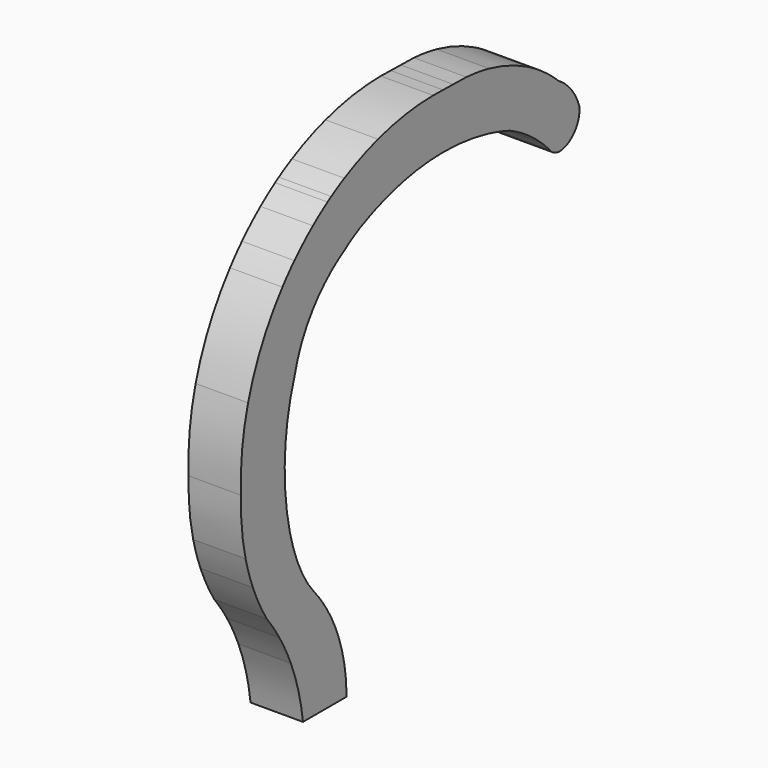
from build123d import *

# Parameters (mm, degrees)
F0_W     = 7.3179761397
F0_H     = 0.852221109
F2_DEPTH = 8


with BuildPart() as f2:
    # F0 (on Right) → F2 (new body)
    with BuildSketch(Plane.YZ):
        with BuildLine():
            Line((-10.1888944263, 53.9168607201), (-5.7503742038, 53.9168607201))
            ThreePointArc((-5.7503742038, 53.9168607201), (-4.3894384073, 57.8607093725), (-2.2639043723, 61.4507223949))
            Line((-2.2639043723, 61.4507223949), (-2.2639043723, 66.7907201963))
            add(Edge.make_bspline(
                [(-10.1888944263, 53.9168607201), (-8.3345715025, 58.6916164824), (-4.5405432149, 63.9948893867), (-2.2639043723, 66.7907201963)],
                knots=[0.4485191098, 0.4485191098, 0.4485191098, 0.4485191098, 0.5436368318, 0.5436368318, 0.5436368318, 0.5436368318], degree=3))
        make_face()
        with BuildLine():
            add(Edge.make_bspline(
                [(-5.7503742038, 53.9168607201), (-7.6414888716, 48.4947767316), (-7.6414888716, 42.0372994525)],
                knots=[4.1382491567, 4.1382491567, 4.1382491567, 4.7123889804, 4.7123889804, 4.7123889804], degree=2, weights=[1, 0.9590776261, 1]))
            Line((-5.7503742038, 53.9168607201), (-10.1888944263, 53.9168607201))
            add(Edge.make_bspline(
                [(-11.7964888716, 42.0372994525), (-11.953273607, 45.832214532), (-11.8401507048, 49.6649877966), (-10.1888944263, 53.9168607201)],
                knots=[0.3638177163, 0.3638177163, 0.3638177163, 0.3638177163, 0.4485191098, 0.4485191098, 0.4485191098, 0.4485191098], degree=3))
            Line((-11.7964888716, 42.0372994525), (-7.6414888716, 42.0372994525))
        make_face()
        with BuildLine():
            add(Edge.make_bspline(
                [(-7.6414888716, 42.0372994525), (-7.6414888716, 37.3930199427), (-6.6239046752, 33.1494348573)],
                knots=[4.7123889804, 4.7123889804, 4.7123889804, 5.1308312404, 5.1308312404, 5.1308312404], degree=2, weights=[1, 0.9781929812, 1]))
            Line((-7.6414888716, 42.0372994525), (-11.7964888716, 42.0372994525))
            add(Edge.make_bspline(
                [(-10.8578113303, 33.1494348573), (-11.3245159446, 35.5121547718), (-11.6611145328, 38.7606149052), (-11.7964888716, 42.0372994525)],
                knots=[0.2906830765, 0.2906830765, 0.2906830765, 0.2906830765, 0.3638177163, 0.3638177163, 0.3638177163, 0.3638177163], degree=3))
            Line((-10.8578113303, 33.1494348573), (-6.6239046752, 33.1494348573))
        make_face()
        with BuildLine():
            Line((-2.2639043723, 66.7907201963), (-2.2639043723, 61.4507223949))
            ThreePointArc((-2.2639043723, 61.4507223949), (-0.6270073096, 63.4042822038), (1.237973472, 65.1414277376))
            Line((1.237973472, 65.1414277376), (1.237973472, 66.7907201963))
            Line((1.237973472, 66.7907201963), (-2.2639043723, 66.7907201963))
        make_face()
        with BuildLine():
            add(Edge.make_bspline(
                [(-11.7964888716, 42.0372994525), (-11.953273607, 45.832214532), (-11.8401507048, 49.6649877966), (-10.1888944263, 53.9168607201)],
                knots=[0.3638177163, 0.3638177163, 0.3638177163, 0.3638177163, 0.4485191098, 0.4485191098, 0.4485191098, 0.4485191098], degree=3))
            Line((-10.1888944263, 53.9168607201), (-14.6274146488, 53.9168607201))
            ThreePointArc((-14.6274146488, 53.9168607201), (-15.7735164452, 48.0310330528), (-15.9514888716, 42.0372994525))
            Line((-15.9514888716, 42.0372994525), (-11.7964888716, 42.0372994525))
        make_face()
        with BuildLine():
            Line((-14.6274146488, 53.9168607201), (-10.1888944263, 53.9168607201))
            add(Edge.make_bspline(
                [(-10.1888944263, 53.9168607201), (-8.3345715025, 58.6916164824), (-4.5405432149, 63.9948893867), (-2.2639043723, 66.7907201963)],
                knots=[0.4485191098, 0.4485191098, 0.4485191098, 0.4485191098, 0.5436368318, 0.5436368318, 0.5436368318, 0.5436368318], degree=3))
            Line((-2.2639043723, 66.7907201963), (-8.0789732143, 66.7907201963))
            ThreePointArc((-8.0789732143, 66.7907201963), (-11.9890354693, 60.6772188038), (-14.6274146488, 53.9168607201))
        make_face()
        with BuildLine():
            add(Edge.make_bspline(
                [(-6.6239046752, 33.1494348573), (-6.0548250045, 30.7762277933), (-5.2018884672, 28.7161691389)],
                knots=[5.1308312404, 5.1308312404, 5.1308312404, 5.3672118342, 5.3672118342, 5.3672118342], degree=2, weights=[1, 0.9930236536, 1]))
            Line((-6.6239046752, 33.1494348573), (-10.8578113303, 33.1494348573))
            add(Edge.make_bspline(
                [(-9.4522823352, 28.7161691389), (-10.1167744763, 30.2015624686), (-10.5211448069, 31.4450405251), (-10.8578113303, 33.1494348573)],
                knots=[0.2379259703, 0.2379259703, 0.2379259703, 0.2379259703, 0.2906830765, 0.2906830765, 0.2906830765, 0.2906830765], degree=3))
            Line((-9.4522823352, 28.7161691389), (-5.2018884672, 28.7161691389))
        make_face()
        with BuildLine():
            add(Edge.make_bspline(
                [(-10.8578113303, 33.1494348573), (-11.3245159446, 35.5121547718), (-11.6611145328, 38.7606149052), (-11.7964888716, 42.0372994525)],
                knots=[0.2906830765, 0.2906830765, 0.2906830765, 0.2906830765, 0.3638177163, 0.3638177163, 0.3638177163, 0.3638177163], degree=3))
            Line((-11.7964888716, 42.0372994525), (-15.9514888716, 42.0372994525))
            ThreePointArc((-15.9514888716, 42.0372994525), (-15.825139965, 37.5640044352), (-15.0917179854, 33.1494348573))
            Line((-15.0917179854, 33.1494348573), (-10.8578113303, 33.1494348573))
        make_face()
        with BuildLine():
            Line((1.237973472, 66.7907201963), (1.237973472, 65.1414277376))
            ThreePointArc((1.237973472, 65.1414277376), (2.366186126, 66.0058819106), (3.5511644697, 66.7907201963))
            Line((3.5511644697, 66.7907201963), (1.237973472, 66.7907201963))
        make_face()
        with BuildLine():
            add(Edge.make_bspline(
                [(-2.2639043723, 66.7907201963), (-1.2992613055, 67.9753520122), (-0.6070401721, 68.7098144761), (0.2691752969, 69.4241264728)],
                knots=[0.5436368318, 0.5436368318, 0.5436368318, 0.5436368318, 0.5839395136, 0.5839395136, 0.5839395136, 0.5839395136], degree=3))
            Line((-2.2639043723, 66.7907201963), (1.237973472, 66.7907201963))
            Line((1.237973472, 66.7907201963), (1.237973472, 69.4241264728))
            Line((1.237973472, 69.4241264728), (0.2691752969, 69.4241264728))
        make_face()
        with BuildLine():
            Line((-8.0789732143, 66.7907201963), (-2.2639043723, 66.7907201963))
            Line((-2.2639043723, 66.7907201963), (-2.2639043723, 69.4241264728))
            Line((-2.2639043723, 69.4241264728), (-5.7937727942, 69.4241264728))
            ThreePointArc((-5.7937727942, 69.4241264728), (-6.9674844154, 68.1344209955), (-8.0789732143, 66.7907201963))
        make_face()
        with BuildLine():
            Line((-2.2639043723, 69.4241264728), (-2.2639043723, 66.7907201963))
            add(Edge.make_bspline(
                [(-2.2639043723, 66.7907201963), (-1.2992613055, 67.9753520122), (-0.6070401721, 68.7098144761), (0.2691752969, 69.4241264728)],
                knots=[0.5436368318, 0.5436368318, 0.5436368318, 0.5436368318, 0.5839395136, 0.5839395136, 0.5839395136, 0.5839395136], degree=3))
            Line((0.2691752969, 69.4241264728), (-2.2639043723, 69.4241264728))
        make_face()
        with BuildLine():
            add(Edge.make_bspline(
                [(-5.2018884672, 28.7161691389), (-3.8937096158, 25.55658452), (-2.0688837208, 23.4551739871)],
                knots=[5.3672118342, 5.3672118342, 5.3672118342, 5.727505896, 5.727505896, 5.727505896], degree=2, weights=[1, 0.9838173593, 1]))
            Line((-5.2018884672, 28.7161691389), (-9.4522823352, 28.7161691389))
            add(Edge.make_bspline(
                [(-6.5688837208, 23.4551739871), (-7.6073097342, 25.0299710332), (-8.6975714446, 27.0291025005), (-9.4522823352, 28.7161691389)],
                knots=[0.1780059801, 0.1780059801, 0.1780059801, 0.1780059801, 0.2379259703, 0.2379259703, 0.2379259703, 0.2379259703], degree=3))
            Line((-6.5688837208, 23.4551739871), (-2.0688837208, 23.4551739871))
        make_face()
        with BuildLine():
            add(Edge.make_bspline(
                [(-9.4522823352, 28.7161691389), (-10.1167744763, 30.2015624686), (-10.5211448069, 31.4450405251), (-10.8578113303, 33.1494348573)],
                knots=[0.2379259703, 0.2379259703, 0.2379259703, 0.2379259703, 0.2906830765, 0.2906830765, 0.2906830765, 0.2906830765], degree=3))
            Line((-10.8578113303, 33.1494348573), (-15.0917179854, 33.1494348573))
            ThreePointArc((-15.0917179854, 33.1494348573), (-14.475702404, 30.9082045202), (-13.7026762032, 28.7161691389))
            Line((-13.7026762032, 28.7161691389), (-9.4522823352, 28.7161691389))
        make_face()
        with BuildLine():
            Line((1.237973472, 66.7907201963), (3.5511644697, 66.7907201963))
            ThreePointArc((3.5511644697, 66.7907201963), (5.8260641015, 68.2586124131), (8.2697197383, 69.4241264728))
            Line((8.2697197383, 69.4241264728), (1.237973472, 69.4241264728))
            Line((1.237973472, 69.4241264728), (1.237973472, 66.7907201963))
        make_face()
        with BuildLine():
            Line((-2.2639043723, 72.6719278562), (-2.2639043723, 69.4241264728))
            Line((-2.2639043723, 69.4241264728), (0.2691752969, 69.4241264728))
            add(Edge.make_bspline(
                [(0.2691752969, 69.4241264728), (0.5652336546, 69.6654803909), (0.8822977177, 69.9045338318), (1.237973472, 70.1578745178)],
                knots=[0.5839395136, 0.5839395136, 0.5839395136, 0.5839395136, 0.5975571068, 0.5975571068, 0.5975571068, 0.5975571068], degree=3))
            Line((1.237973472, 70.1578745177), (1.237973472, 74.7149176101))
            Line((1.237973472, 74.7149176101), (0.5268579819, 74.7149176101))
            ThreePointArc((0.5268579819, 74.7149176101), (-0.8924649684, 73.7261276448), (-2.2639043723, 72.6719278562))
        make_face()
        with BuildLine():
            Line((-5.7937727942, 69.4241264728), (-2.2639043723, 69.4241264728))
            Line((-2.2639043723, 69.4241264728), (-2.2639043723, 72.6719278562))
            ThreePointArc((-2.2639043723, 72.6719278562), (-4.0816510588, 71.1054263302), (-5.7937727942, 69.4241264728))
        make_face()
        with BuildLine():
            add(Edge.make_bspline(
                [(0.2691752969, 69.4241264728), (0.5652336546, 69.6654803909), (0.8822977177, 69.9045338318), (1.237973472, 70.1578745178)],
                knots=[0.5839395136, 0.5839395136, 0.5839395136, 0.5839395136, 0.5975571068, 0.5975571068, 0.5975571068, 0.5975571068], degree=3))
            Line((0.2691752969, 69.4241264728), (1.237973472, 69.4241264728))
            Line((1.237973472, 69.4241264728), (1.237973472, 70.1578745177))
        make_face()
        with BuildLine():
            ThreePointArc((0.4889115668, 19.9429222314), (-0.7147477725, 21.7538403606), (-2.0688837208, 23.4551739871))
            Line((-2.0688837208, 23.4551739871), (-6.5688837208, 23.4551739871))
            add(Edge.make_bspline(
                [(-4.0796691275, 19.9429222314), (-4.8467986494, 21.0916706181), (-5.6892435404, 22.121179326), (-6.5688837208, 23.4551739871)],
                knots=[0.127248362, 0.127248362, 0.127248362, 0.127248362, 0.1780059801, 0.1780059801, 0.1780059801, 0.1780059801], degree=3))
            Line((-4.0796691275, 19.9429222314), (0.4889115668, 19.9429222314))
        make_face()
        with BuildLine():
            add(Edge.make_bspline(
                [(-6.5688837208, 23.4551739871), (-7.6073097342, 25.0299710332), (-8.6975714446, 27.0291025005), (-9.4522823352, 28.7161691389)],
                knots=[0.1780059801, 0.1780059801, 0.1780059801, 0.1780059801, 0.2379259703, 0.2379259703, 0.2379259703, 0.2379259703], degree=3))
            Line((-9.4522823352, 28.7161691389), (-13.7026762032, 28.7161691389))
            ThreePointArc((-13.7026762032, 28.7161691389), (-12.5038516774, 26.0265617582), (-11.0688837208, 23.4551739871))
            Line((-11.0688837208, 23.4551739871), (-6.5688837208, 23.4551739871))
        make_face()
        with BuildLine():
            Line((1.237973472, 69.4241264728), (8.2697197383, 69.4241264728))
            ThreePointArc((8.2697197383, 69.4241264728), (9.1992306977, 69.8164897066), (10.1393910192, 70.1826018489))
            Line((10.1393910192, 70.1826018489), (10.1393910192, 74.7149176101))
            add(Edge.make_bspline(
                [(1.237973472, 70.1578745178), (3.2585532739, 71.5970928701), (6.5252601055, 73.4974078941), (10.1393910192, 74.7149176101)],
                knots=[0.5975571068, 0.5975571068, 0.5975571068, 0.5975571068, 0.6749181117, 0.6749181117, 0.6749181117, 0.6749181117], degree=3))
            Line((1.237973472, 70.1578745177), (1.237973472, 69.4241264728))
        make_face()
        with BuildLine():
            Line((1.237973472, 74.7149176101), (1.237973472, 70.1578745177))
            add(Edge.make_bspline(
                [(1.237973472, 70.1578745178), (3.2585532739, 71.5970928701), (6.5252601055, 73.4974078941), (10.1393910192, 74.7149176101)],
                knots=[0.5975571068, 0.5975571068, 0.5975571068, 0.5975571068, 0.6749181117, 0.6749181117, 0.6749181117, 0.6749181117], degree=3))
            Line((10.1393910192, 74.7149176101), (1.237973472, 74.7149176101))
        make_face()
        with BuildLine():
            ThreePointArc((2.5784133808, 15.6048506081), (1.6366902241, 17.8235113891), (0.4889115668, 19.9429222314))
            Line((0.4889115668, 19.9429222314), (-4.0796691275, 19.9429222314))
            add(Edge.make_bspline(
                [(-1.9430062522, 15.6048506081), (-2.5381682165, 17.3739492027), (-3.2666174927, 18.7254071612), (-4.0796691275, 19.9429222314)],
                knots=[0.0734522777, 0.0734522777, 0.0734522777, 0.0734522777, 0.127248362, 0.127248362, 0.127248362, 0.127248362], degree=3))
            Line((-1.9430062522, 15.6048506081), (2.5784133808, 15.6048506081))
        make_face()
        with BuildLine():
            add(Edge.make_bspline(
                [(-4.0796691275, 19.9429222314), (-4.8467986494, 21.0916706181), (-5.6892435404, 22.121179326), (-6.5688837208, 23.4551739871)],
                knots=[0.127248362, 0.127248362, 0.127248362, 0.127248362, 0.1780059801, 0.1780059801, 0.1780059801, 0.1780059801], degree=3))
            Line((-6.5688837208, 23.4551739871), (-11.0688837208, 23.4551739871))
            ThreePointArc((-11.0688837208, 23.4551739871), (-9.80227604, 21.7378435208), (-8.6482498217, 19.9429222314))
            Line((-8.6482498217, 19.9429222314), (-4.0796691275, 19.9429222314))
        make_face()
        with BuildLine():
            Line((10.1393910192, 74.7149176101), (10.1393910192, 70.1826018489))
            ThreePointArc((10.1393910192, 70.1826018489), (16.2528045864, 71.8676558179), (22.5672341212, 72.4517893404))
            Line((22.5672341212, 72.4517893404), (22.5672341212, 76.6135193731))
            add(Edge.make_bspline(
                [(10.1393910192, 74.7149176101), (14.1917188378, 76.0800448315), (18.6808252051, 76.5867551297), (22.5672341212, 76.6135193731)],
                knots=[0.6749181117, 0.6749181117, 0.6749181117, 0.6749181117, 0.7616587859, 0.7616587859, 0.7616587859, 0.7616587859], degree=3))
        make_face()
        with BuildLine():
            ThreePointArc((1.237973472, 75.1743212979), (0.8810985763, 74.9466582845), (0.5268579819, 74.7149176101))
            Line((0.5268579819, 74.7149176101), (1.237973472, 74.7149176101))
            Line((1.237973472, 74.7149176101), (1.237973472, 75.1743212979))
        make_face()
        with BuildLine():
            Line((1.237973472, 75.1743212979), (1.237973472, 74.7149176101))
            Line((1.237973472, 74.7149176101), (10.1393910192, 74.7149176101))
            Line((10.1393910192, 74.7149176101), (10.1393910192, 76.6135193731))
            Line((10.1393910192, 76.6135193731), (3.7337425961, 76.6135193731))
            ThreePointArc((3.7337425961, 76.6135193731), (2.4718112827, 75.918279351), (1.237973472, 75.1743212979))
        make_face()
        with BuildLine():
            Line((10.1393910192, 76.6135193731), (10.1393910192, 74.7149176101))
            add(Edge.make_bspline(
                [(10.1393910192, 74.7149176101), (14.1917188378, 76.0800448315), (18.6808252051, 76.5867551297), (22.5672341212, 76.6135193731)],
                knots=[0.6749181117, 0.6749181117, 0.6749181117, 0.6749181117, 0.7616587859, 0.7616587859, 0.7616587859, 0.7616587859], degree=3))
            Line((22.5672341212, 76.6135193731), (10.1393910192, 76.6135193731))
        make_face()
        with BuildLine():
            ThreePointArc((4.152898933, 6.8011660784), (3.7561793875, 11.2728510531), (2.5784133808, 15.6048506081))
            Line((2.5784133808, 15.6048506081), (-1.9430062522, 15.6048506081))
            add(Edge.make_bspline(
                [(-0.002101067, 6.8011660784), (-0.5662415412, 9.9952594602), (-1.1303820154, 13.189352842), (-1.9430062522, 15.6048506081)],
                knots=[0, 0, 0, 0, 0.0734522777, 0.0734522777, 0.0734522777, 0.0734522777], degree=3))
            Line((-0.002101067, 6.8011660784), (4.152898933, 6.8011660784))
        make_face()
        with BuildLine():
            add(Edge.make_bspline(
                [(-1.9430062522, 15.6048506081), (-2.5381682165, 17.3739492027), (-3.2666174927, 18.7254071612), (-4.0796691275, 19.9429222314)],
                knots=[0.0734522777, 0.0734522777, 0.0734522777, 0.0734522777, 0.127248362, 0.127248362, 0.127248362, 0.127248362], degree=3))
            Line((-4.0796691275, 19.9429222314), (-8.6482498217, 19.9429222314))
            ThreePointArc((-8.6482498217, 19.9429222314), (-7.4771524819, 17.8137490419), (-6.4644258852, 15.6048506081))
            Line((-6.4644258852, 15.6048506081), (-1.9430062522, 15.6048506081))
        make_face()
        with BuildLine():
            Line((22.5672341212, 76.6135193731), (22.5672341212, 72.4517893404))
            ThreePointArc((22.5672341212, 72.4517893404), (26.9794357563, 72.1971647924), (31.3270061461, 71.4028168618))
            Line((31.3270061461, 71.4028168618), (31.3270061461, 72.690683065))
            Line((31.3270061461, 72.690683065), (31.3270061461, 75.761298264))
            add(Edge.make_bspline(
                [(23.2156569251, 76.6135193731), (26.1977321335, 76.5927510585), (28.8283393897, 76.2847039305), (31.3270061461, 75.761298264)],
                knots=[0.7665245528, 0.7665245528, 0.7665245528, 0.7665245528, 0.8342341594, 0.8342341594, 0.8342341594, 0.8342341594], degree=3))
            Line((23.2156569251, 76.6135193731), (22.5672341212, 76.6135193731))
        make_face()
        with BuildLine():
            Line((3.7337425961, 76.6135193731), (10.1393910192, 76.6135193731))
            Line((10.1393910192, 76.6135193731), (10.1393910192, 79.2472333713))
            ThreePointArc((10.1393910192, 79.2472333713), (6.8746578417, 78.0809496958), (3.7337425961, 76.6135193731))
        make_face()
        with BuildLine():
            Line((10.1393910192, 79.2472333713), (10.1393910192, 76.6135193731))
            Line((10.1393910192, 76.6135193731), (22.5672341212, 76.6135193731))
            Line((22.5672341212, 76.6135193731), (22.5672341212, 80.816700989))
            Line((22.5672341212, 80.816700989), (20.6527994041, 80.8529768738))
            ThreePointArc((20.6527994041, 80.8529768738), (15.3379592409, 80.4307432513), (10.1393910192, 79.2472333713))
        make_face()
        with BuildLine():
            Line((22.5672341212, 80.816700989), (22.5672341212, 76.6135193731))
            add(Edge.make_bspline(
                [(22.5672341212, 76.6135193731), (22.7852444149, 76.6150207283), (23.0013581932, 76.6150118316), (23.2156569251, 76.6135193731)],
                knots=[0.7616587859, 0.7616587859, 0.7616587859, 0.7616587859, 0.7665245528, 0.7665245528, 0.7665245528, 0.7665245528], degree=3))
            Line((23.2156569251, 76.6135193731), (31.3270061461, 76.6135193731))
            Line((31.3270061461, 76.6135193731), (31.3270061461, 80.1197796662))
            ThreePointArc((31.3270061461, 80.1197796662), (29.1770875592, 80.5100007635), (27.0034147385, 80.7326415141))
            Line((27.0034147385, 80.7326415141), (24.5007061931, 80.7800643727))
            Line((24.5007061931, 80.7800643727), (22.5672341212, 80.816700989))
        make_face()
        with BuildLine():
            add(Edge.make_bspline(
                [(-0.002101067, 6.8011660784), (-0.5662415412, 9.9952594602), (-1.1303820154, 13.189352842), (-1.9430062522, 15.6048506081)],
                knots=[0, 0, 0, 0, 0.0734522777, 0.0734522777, 0.0734522777, 0.0734522777], degree=3))
            Line((-1.9430062522, 15.6048506081), (-6.4644258852, 15.6048506081))
            ThreePointArc((-6.4644258852, 15.6048506081), (-5.008614741, 11.2821973774), (-4.157101067, 6.8011660784))
            Line((-4.157101067, 6.8011660784), (-0.002101067, 6.8011660784))
        make_face()
        with BuildLine():
            Line((31.3270061461, 72.690683065), (31.3270061461, 71.4028168618))
            ThreePointArc((31.3270061461, 71.4028168618), (33.333189747, 70.8449262382), (35.3036885535, 70.1717627798))
            ThreePointArc((35.3036885535, 70.1717627798), (37.0126027179, 69.2615348872), (38.6449822857, 68.2202667256))
            Line((38.6449822857, 68.2202667256), (38.6449822857, 72.7516210723))
            Line((38.6449822857, 72.7516210723), (31.3270061461, 72.690683065))
        make_face()
        with BuildLine():
            Line((31.3270061461, 76.6135193731), (23.2156569251, 76.6135193731))
            add(Edge.make_bspline(
                [(23.2156569251, 76.6135193731), (26.1977321335, 76.5927510585), (28.8283393897, 76.2847039305), (31.3270061461, 75.761298264)],
                knots=[0.7665245528, 0.7665245528, 0.7665245528, 0.7665245528, 0.8342341594, 0.8342341594, 0.8342341594, 0.8342341594], degree=3))
            Line((31.3270061461, 75.761298264), (31.3270061461, 76.6135193731))
        make_face()
        with BuildLine():
            Line((31.3270061461, 75.761298264), (31.3270061461, 72.690683065))
            Line((31.3270061461, 72.690683065), (38.6449822857, 72.7516210723))
            Line((38.6449822857, 72.7516210723), (38.6449822857, 72.804503681))
            add(Edge.make_bspline(
                [(31.3270061461, 75.761298264), (33.8632565179, 75.2300198081), (36.2635673813, 74.4768554728), (38.6449822857, 72.804503681)],
                knots=[0.8342341594, 0.8342341594, 0.8342341594, 0.8342341594, 0.9029622179, 0.9029622179, 0.9029622179, 0.9029622179], degree=3))
        make_face()
        with BuildLine():
            Line((31.3270061461, 80.1197796662), (31.3270061461, 76.6135193731))
            Line((31.3270061461, 76.6135193731), (38.6449822857, 76.6135193731))
            Line((38.6449822857, 76.6135193731), (38.6449822857, 77.3887406365))
            ThreePointArc((38.6449822857, 77.3887406365), (35.0809806575, 79.0087817843), (31.3270061461, 80.1197796662))
        make_face()
        with Locations((34.9859942159, 76.1874088185)):
            Rectangle(F0_W, F0_H)
        with BuildLine():
            Line((38.6449822857, 75.761298264), (31.3270061461, 75.761298264))
            add(Edge.make_bspline(
                [(31.3270061461, 75.761298264), (33.8632565179, 75.2300198081), (36.2635673813, 74.4768554728), (38.6449822857, 72.804503681)],
                knots=[0.8342341594, 0.8342341594, 0.8342341594, 0.8342341594, 0.9029622179, 0.9029622179, 0.9029622179, 0.9029622179], degree=3))
            Line((38.6449822857, 72.804503681), (38.6449822857, 75.761298264))
        make_face()
        with BuildLine():
            Line((38.6449822857, 72.7516210723), (38.6449822857, 68.2202667256))
            ThreePointArc((38.6449822857, 68.2202667256), (39.3339273149, 67.7240475044), (40.0054134636, 67.2044465799))
            Line((40.0054134636, 67.2044465799), (44.2810582439, 67.2044465799))
            add(Edge.make_bspline(
                [(38.7189835451, 72.7522372931), (41.0830829077, 71.0729861649), (43.413637043, 68.5097934745), (44.2810582439, 67.2044465799)],
                knots=[0.9036741885, 0.9036741885, 0.9036741885, 0.9036741885, 0.9719182271, 0.9719182271, 0.9719182271, 0.9719182271], degree=3))
            Line((38.7189835451, 72.7522372931), (38.6449822857, 72.7516210723))
        make_face()
        with BuildLine():
            Line((38.6449822857, 77.3887406365), (38.6449822857, 76.6135193731))
            Line((38.6449822857, 76.6135193731), (39.9877868127, 76.6135193731))
            ThreePointArc((39.9877868127, 76.6135193731), (39.3217119492, 77.010357895), (38.6449822857, 77.3887406365))
        make_face()
        with BuildLine():
            Line((39.9877868127, 76.6135193731), (38.6449822857, 76.6135193731))
            Line((38.6449822857, 76.6135193731), (38.6449822857, 75.761298264))
            Line((38.6449822857, 75.761298264), (41.2922999092, 75.761298264))
            ThreePointArc((41.2922999092, 75.761298264), (40.6459290143, 76.1964181141), (39.9877868127, 76.6135193731))
        make_face()
        with BuildLine():
            Line((41.2922999092, 75.761298264), (38.6449822857, 75.761298264))
            Line((38.6449822857, 75.761298264), (38.6449822857, 72.804503681))
            add(Edge.make_bspline(
                [(38.6449822857, 72.804503681), (38.6696519411, 72.7871793827), (38.6943195687, 72.7697564427), (38.7189835451, 72.7522372931)],
                knots=[0.9029622179, 0.9029622179, 0.9029622179, 0.9029622179, 0.9036741885, 0.9036741885, 0.9036741885, 0.9036741885], degree=3))
            Line((38.7189835451, 72.7522372931), (44.8563766883, 72.803344389))
            Line((44.8563766883, 72.803344389), (44.8563766883, 72.8972181129))
            ThreePointArc((44.8563766883, 72.8972181129), (44.7546139615, 72.9626942681), (44.6519926928, 73.0268164536))
            ThreePointArc((44.6519926928, 73.0268164536), (43.0247143735, 74.4586445772), (41.2922999092, 75.761298264))
        make_face()
        with BuildLine():
            Line((44.2810582439, 67.2044465799), (40.0054134636, 67.2044465799))
            ThreePointArc((40.0054134636, 67.2044465799), (40.7024608637, 66.6243204625), (41.3777458899, 66.0190011059))
            Line((41.3777458899, 66.0190011059), (44.2810582439, 66.0190011059))
            Line((44.2810582439, 66.0190011059), (44.2810582439, 67.2044465799))
        make_face()
        with BuildLine():
            Line((44.8563766883, 72.803344389), (38.7189835451, 72.7522372931))
            add(Edge.make_bspline(
                [(38.7189835451, 72.7522372931), (41.0830829077, 71.0729861649), (43.413637043, 68.5097934745), (44.2810582439, 67.2044465799)],
                knots=[0.9036741885, 0.9036741885, 0.9036741885, 0.9036741885, 0.9719182271, 0.9719182271, 0.9719182271, 0.9719182271], degree=3))
            Line((44.2810582439, 67.2044465799), (44.8563766883, 67.2044465799))
            Line((44.8563766883, 67.2044465799), (44.8563766883, 72.803344389))
        make_face()
        with BuildLine():
            Line((44.2810582439, 66.0190011059), (41.3777458899, 66.0190011059))
            ThreePointArc((41.3777458899, 66.0190011059), (42.1468438935, 65.2719221816), (42.8828000164, 64.4921739894))
            ThreePointArc((42.8828000164, 64.4921739894), (42.8721611441, 64.5060256939), (42.8616194891, 64.5199515271))
            Line((42.8616194891, 64.5199515271), (43.1128631572, 64.2339614732))
            ThreePointArc((43.1128631572, 64.2339614732), (43.653215449, 63.8329981426), (44.2810582439, 63.5909948022))
            Line((44.2810582439, 63.5909948022), (44.2810582439, 66.0190011059))
        make_face()
        with BuildLine():
            add(Edge.make_bspline(
                [(44.2810582439, 67.2044465799), (44.63799382, 66.667308745), (44.7471852541, 66.3431549254), (44.8563766883, 66.0190011059)],
                knots=[0.9719182271, 0.9719182271, 0.9719182271, 0.9719182271, 1, 1, 1, 1], degree=3))
            Line((44.2810582439, 67.2044465799), (44.2810582439, 66.0190011059))
            Line((44.2810582439, 66.0190011059), (44.8563766883, 66.0190011059))
        make_face()
        with BuildLine():
            Line((44.8563766883, 67.2044465799), (44.2810582439, 67.2044465799))
            add(Edge.make_bspline(
                [(44.2810582439, 67.2044465799), (44.63799382, 66.667308745), (44.7471852541, 66.3431549254), (44.8563766883, 66.0190011059)],
                knots=[0.9719182271, 0.9719182271, 0.9719182271, 0.9719182271, 1, 1, 1, 1], degree=3))
            Line((44.8563766883, 66.0190011059), (44.8563766883, 67.2044465799))
        make_face()
        with BuildLine():
            Line((44.995594754, 72.804503681), (44.8563766883, 72.803344389))
            Line((44.8563766883, 72.803344389), (44.8563766883, 67.2044465799))
            Line((44.8563766883, 67.2044465799), (48.5567030241, 67.2044465799))
            ThreePointArc((48.5567030241, 67.2044465799), (48.5776505922, 67.6306605106), (48.5547722523, 68.0567751628))
            ThreePointArc((48.5547722523, 68.0567751628), (47.1714888934, 70.7277333316), (44.995594754, 72.804503681))
        make_face()
        with BuildLine():
            Line((44.8563766883, 66.0190011059), (44.2810582439, 66.0190011059))
            Line((44.2810582439, 66.0190011059), (44.2810582439, 63.5909948022))
            ThreePointArc((44.2810582439, 63.5909948022), (44.8744379473, 63.5238298264), (45.4667831786, 63.5995776539))
            ThreePointArc((45.4667831786, 63.5995776539), (47.1450780919, 64.4823835606), (48.2563056132, 66.0190011059))
            Line((48.2563056132, 66.0190011059), (44.8563766883, 66.0190011059))
        make_face()
        with BuildLine():
            Line((48.5567030241, 67.2044465799), (44.8563766883, 67.2044465799))
            Line((44.8563766883, 67.2044465799), (44.8563766883, 66.0190011059))
            Line((44.8563766883, 66.0190011059), (48.2563056132, 66.0190011059))
            ThreePointArc((48.2563056132, 66.0190011059), (48.4503561043, 66.6006115959), (48.5567030241, 67.2044465799))
        make_face()
    extrude(amount=F2_DEPTH)


solid = f2.part
